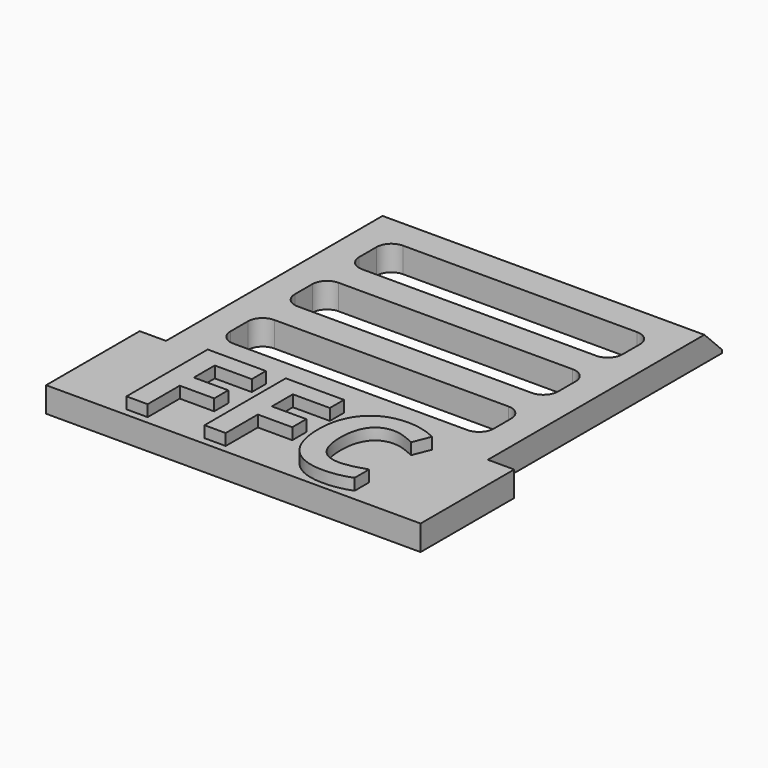
from build123d import *

# Parameters (mm, degrees)
F0_W         = 22
F0_H         = 20
F0_W_2       = 18
F0_H_2       = 3.5
F0_TEXT_SIZE = 9.7222222222
F1_DEPTH     = 1.72
F2_DEPTH     = 2.5
F3_SIZE      = 1.5
F4_R         = 1


# Not quite as in the source:
# - Text() gives the source's letters only with a copy of the font that has no kerning and outlines rounded to 1/6400 em; it was checked with that copy


with BuildPart() as f1:
    # F0 (on Top) → F1 (new body)
    with BuildSketch(Plane.XY):
        Polygon((11, 0), (-11, 0), (-12.8, 0), (-12.8, -8), (12.8, -8), (12.8, 0), align=None)
        Polygon((-6.2571614583, -4.7565104167), (-6.2571614583, -7.5), (-7.7048611111, -7.5), (-7.7048611111, -0.5592447917), (-3.7263454861, -0.5592447917), (-3.7263454861, -1.7654079861), (-6.2571614583, -1.7654079861), (-6.2571614583, -3.5549045139), (-3.9025607639, -3.5549045139), (-3.9025607639, -4.7565104167), align=None, mode=Mode.SUBTRACT)
        Polygon((-0.9205729167, -4.7565104167), (-0.9205729167, -7.5), (-2.3682725694, -7.5), (-2.3682725694, -0.5592447917), (1.6102430556, -0.5592447917), (1.6102430556, -1.7654079861), (-0.9205729167, -1.7654079861), (-0.9205729167, -3.5549045139), (1.4340277778, -3.5549045139), (1.4340277778, -4.7565104167), align=None, mode=Mode.SUBTRACT)
        with BuildLine():
            add(Edge.make_bspline(
                [(6.6901041667, -1.8223741319), (6.2966579861, -1.6848958333), (5.9168836806, -1.6848958333)],
                knots=[0, 0, 0, 1, 1, 1], degree=2))
            add(Edge.make_bspline(
                [(5.9168836806, -1.6848958333), (5.0859375, -1.6848958333), (4.6302083333, -2.3092447917)],
                knots=[0, 0, 0, 1, 1, 1], degree=2))
            add(Edge.make_bspline(
                [(4.6302083333, -2.3092447917), (4.1744791667, -2.93359375), (4.1744791667, -4.0486111111)],
                knots=[0, 0, 0, 1, 1, 1], degree=2))
            add(Edge.make_bspline(
                [(4.1744791667, -4.0486111111), (4.1744791667, -6.3697916667), (5.9168836806, -6.3697916667)],
                knots=[0, 0, 0, 1, 1, 1], degree=2))
            add(Edge.make_bspline(
                [(5.9168836806, -6.3697916667), (6.6475694444, -6.3697916667), (7.6866319444, -6.0052083333)],
                knots=[0, 0, 0, 1, 1, 1], degree=2))
            Line((7.6866319444, -6.0052083333), (7.6866319444, -7.2387152778))
            add(Edge.make_bspline(
                [(7.6866319444, -7.2387152778), (6.8328993056, -7.595703125), (5.7786458333, -7.595703125)],
                knots=[0, 0, 0, 1, 1, 1], degree=2))
            add(Edge.make_bspline(
                [(5.7786458333, -7.595703125), (4.2641059028, -7.595703125), (3.4620225694, -6.6766493056)],
                knots=[0, 0, 0, 1, 1, 1], degree=2))
            add(Edge.make_bspline(
                [(3.4620225694, -6.6766493056), (2.6599392361, -5.7575954861), (2.6599392361, -4.0394965278)],
                knots=[0, 0, 0, 1, 1, 1], degree=2))
            add(Edge.make_bspline(
                [(2.6599392361, -4.0394965278), (2.6599392361, -2.9563802083), (3.0541449653, -2.1421440972)],
                knots=[0, 0, 0, 1, 1, 1], degree=2))
            add(Edge.make_bspline(
                [(3.0541449653, -2.1421440972), (3.4483506944, -1.3279079861), (4.1866319444, -0.8942057292)],
                knots=[0, 0, 0, 1, 1, 1], degree=2))
            add(Edge.make_bspline(
                [(4.1866319444, -0.8942057292), (4.9249131944, -0.4605034722), (5.9168836806, -0.4605034722)],
                knots=[0, 0, 0, 1, 1, 1], degree=2))
            add(Edge.make_bspline(
                [(5.9168836806, -0.4605034722), (6.9270833333, -0.4605034722), (7.9479166667, -0.9481336806)],
                knots=[0, 0, 0, 1, 1, 1], degree=2))
            Line((7.9479166667, -0.9481336806), (7.4739583333, -2.1451822917))
            add(Edge.make_bspline(
                [(7.4739583333, -2.1451822917), (7.0835503472, -1.9598524306), (6.6901041667, -1.8223741319)],
                knots=[0, 0, 0, 1, 1, 1], degree=2))
        make_face(mode=Mode.SUBTRACT)
        with Locations((0, 10)):
            Rectangle(F0_W, F0_H)
        with Locations((0, 3.75)):
            Rectangle(F0_W_2, F0_H_2, mode=Mode.SUBTRACT)
        with Locations((0, 9.25)):
            Rectangle(F0_W_2, F0_H_2, mode=Mode.SUBTRACT)
        with Locations((0, 14.75)):
            Rectangle(F0_W_2, F0_H_2, mode=Mode.SUBTRACT)
        with Locations((-8.5783420139, -7.5)):
            Text('FFC', F0_TEXT_SIZE, font='Open Sans', font_style=FontStyle.BOLD, text_align=(TextAlign.LEFT, TextAlign.BOTTOM))
    extrude(amount=F1_DEPTH)

    # F0 (on Top) → F2 (join)
    with BuildSketch(Plane.XY):
        with Locations((-8.5783420139, -7.5)):
            Text('FFC', F0_TEXT_SIZE, font='Open Sans', font_style=FontStyle.BOLD, text_align=(TextAlign.LEFT, TextAlign.BOTTOM))
    extrude(amount=F2_DEPTH)

    # F3
    f3_edges = [f1.edges().sort_by_distance(p)[0] for p in [
        (0, 20, 1.72),
    ]]
    chamfer(f3_edges, length=F3_SIZE)

    # F4
    f4_edges = [f1.edges().sort_by_distance(p)[0] for p in [
        (-9, 16.5, 0.86),
        (9, 16.5, 0.86),
        (9, 11, 0.86),
        (9, 5.5, 0.86),
        (9, 13, 0.86),
        (9, 7.5, 0.86),
        (9, 2, 0.86),
        (-9, 13, 0.86),
        (-9, 7.5, 0.86),
        (-9, 2, 0.86),
        (-9, 5.5, 0.86),
        (-9, 11, 0.86),
    ]]
    fillet(f4_edges, radius=F4_R)


solid = f1.part
